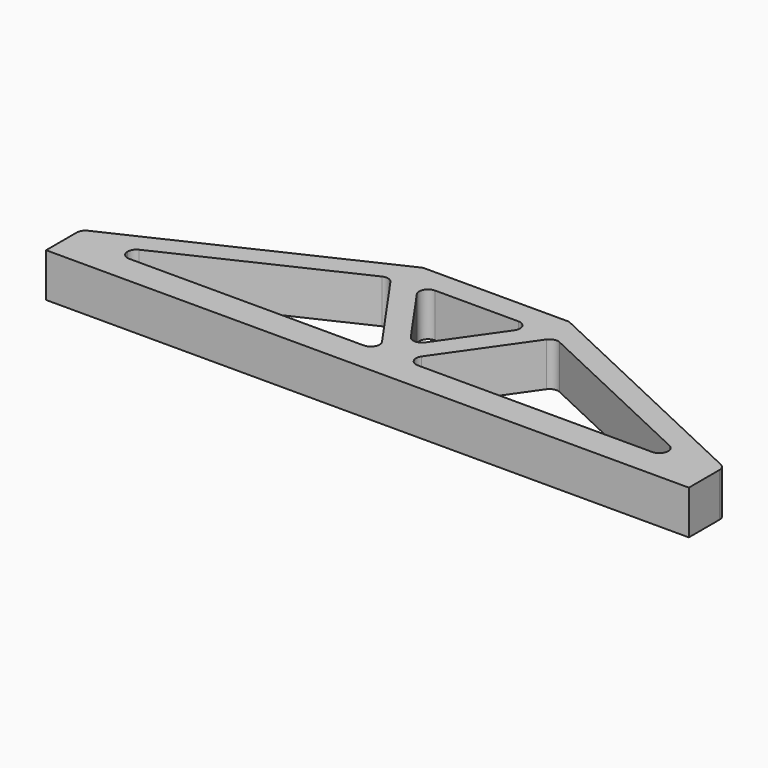
from build123d import *

# Parameters (mm, degrees)
F1_DEPTH = 30
F3_DEPTH = 30.001
F4_R     = 6


with BuildPart() as f1:
    # F0 (on Top) → F1 (new body)
    with BuildSketch(Plane.XY):
        Polygon((-220, -20), (-220, -50), (220, -50), (220, -20), (50, 60), (-50, 60), align=None)
    extrude(amount=F1_DEPTH)

    # F2 (on face) → F3 (cut, through all)
    with BuildSketch(Plane(origin=(0, 0, 0), x_dir=(1, 0, 0), z_dir=(0, 0, -1))):
        Polygon((-185, 30), (-185, 20.1073184365), (-56.2451380356, -40.4832048408), (-7, 30), align=None)
        Polygon((-1.2777449276, 12), (-40, -43.4220933282), (40, -43.4220933282), (1.2777449276, 12), (0, 13.8288009955), align=None)
        Polygon((185, 30), (7, 30), (56.2451380356, -40.4832048408), (185, 20.1073184365), align=None)
    extrude(amount=-F3_DEPTH, mode=Mode.SUBTRACT)

    # F4
    f4_edges = [f1.edges().sort_by_distance(p)[0] for p in [
        (-185, -20.107318, 15),
        (-185, -30, 15),
        (185, -20.107318, 15),
        (185, -30, 15),
        (-50, 60, 15),
        (50, 60, 15),
        (220, -20, 15),
        (-220, -20, 15),
        (-7, -30, 15),
        (7, -30, 15),
        (0, -13.828801, 15),
        (-56.245138, 40.483205, 15),
        (56.245138, 40.483205, 15),
        (40, 43.422093, 15),
        (-40, 43.422093, 15),
    ]]
    fillet(f4_edges, radius=F4_R)


solid = f1.part
